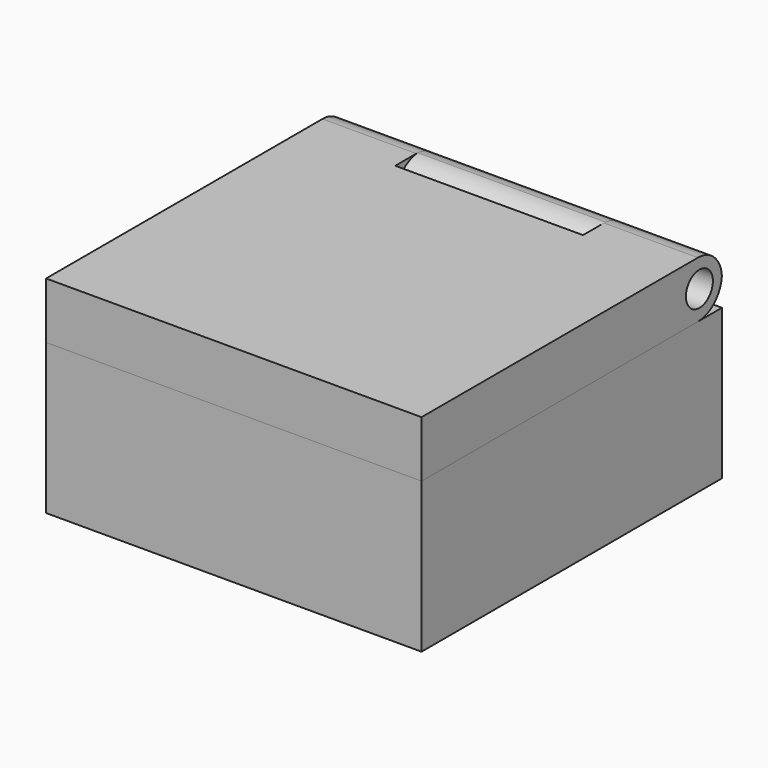
from build123d import *

# Parameters (mm, degrees)
F0_W        = 25.4
F0_H        = 25.4
F1_DEPTH    = 10.16
F2_W        = 17.78
F2_H        = 17.78
F3_DEPTH    = 5.08
F4_W        = 6.35
F4_H        = 3.81
F5_DEPTH    = 3.81
F7_DEPTH    = 3.81
F8_T1_DEPTH = 16.51
F8_T3_DEPTH = 16.51
F9_T1_DEPTH = 22.86
F10_R       = 1.1410136833
F11_DEPTH   = 25.4


# Not quite as in the source:
# - a fillet or chamfer that OpenCascade refuses, or shapes differently, is made with other operations: its cross-section is extruded or revolved along the edge and cut away or added


with BuildPart() as f1:
    # F0 (on Top) → F1 (new body)
    with BuildSketch(Plane.XY):
        with Locations((12.7, 12.7)):
            Rectangle(F0_W, F0_H)
    extrude(amount=F1_DEPTH)

    # F2 (on face) → F3 (cut)
    with BuildSketch(Plane.XY.offset(10.16)):
        with Locations((12.7, 12.7)):
            Rectangle(F2_W, F2_H)
    extrude(amount=-F3_DEPTH, mode=Mode.SUBTRACT)

    # F4 (on face) → F5 (join)
    with BuildSketch(Plane.XY.offset(10.16)):
        with Locations((9.525, 23.495)):
            Rectangle(F4_W, F4_H)
        with Locations((15.875, 23.495)):
            Rectangle(F4_W, F4_H)
    extrude(amount=F5_DEPTH)

    # F9: fillet of radius 2.032 on 2 edges, made by hand

    # F9_s2 → F9_t1 (cut)
    with BuildSketch(Plane.YZ.offset(1.27)):
        with BuildLine():
            ThreePointArc((21.59, 11.938), (22.1851590206, 13.3748409794), (23.622, 13.97))
            Line((23.622, 13.97), (21.59, 13.97))
            Line((21.59, 13.97), (21.59, 11.938))
        make_face()
        with BuildLine():
            ThreePointArc((25.4, 11.938), (24.8048409794, 13.3748409794), (23.368, 13.97))
            Line((23.368, 13.97), (25.4, 13.97))
            Line((25.4, 13.97), (25.4, 11.938))
        make_face()
    extrude(amount=F9_T1_DEPTH, mode=Mode.SUBTRACT)


with BuildPart() as f7:
    # F6 (on face) → F7 (new body)
    with BuildSketch(Plane.XY.offset(10.16)):
        Polygon((3.81, 21.59), (0, 21.59), (0, 0), (25.4, 0), (25.4, 21.59), (21.59, 21.59), (21.59, 3.81), (3.81, 3.81), align=None)
        Polygon((6.35, 21.59), (3.81, 21.59), (3.81, 3.81), (21.59, 3.81), (21.59, 21.59), (19.05, 21.59), align=None)
        Polygon((19.05, 25.4), (19.05, 21.59), (21.59, 21.59), (25.4, 21.59), (25.4, 25.4), align=None)
        Polygon((0, 25.4), (0, 21.59), (3.81, 21.59), (6.35, 21.59), (6.35, 25.4), align=None)
    extrude(amount=F7_DEPTH)

    # F8: fillet of radius 2.032 on 4 edges, made by hand

    # F8_s2 → F8_t1 (cut)
    with BuildSketch(Plane.YZ.offset(-5.08)):
        with BuildLine():
            ThreePointArc((25.4, 12.192), (24.8048409794, 10.7551590206), (23.368, 10.16))
            Line((23.368, 10.16), (25.4, 10.16))
            Line((25.4, 10.16), (25.4, 12.192))
        make_face()
        with BuildLine():
            ThreePointArc((25.4, 11.938), (24.8048409794, 13.3748409794), (23.368, 13.97))
            Line((23.368, 13.97), (25.4, 13.97))
            Line((25.4, 13.97), (25.4, 11.938))
        make_face()
    extrude(amount=F8_T1_DEPTH, mode=Mode.SUBTRACT)

    # F8_s4 → F8_t3 (cut)
    with BuildSketch(Plane.YZ.offset(13.97)):
        with BuildLine():
            ThreePointArc((25.4, 11.938), (24.8048409794, 13.3748409794), (23.368, 13.97))
            Line((23.368, 13.97), (25.4, 13.97))
            Line((25.4, 13.97), (25.4, 11.938))
        make_face()
        with BuildLine():
            ThreePointArc((25.4, 12.192), (24.8048409794, 10.7551590206), (23.368, 10.16))
            Line((23.368, 10.16), (25.4, 10.16))
            Line((25.4, 10.16), (25.4, 12.192))
        make_face()
    extrude(amount=F8_T3_DEPTH, mode=Mode.SUBTRACT)


with BuildPart() as f11_tool:
    # F10 (on face) → F11 (new body)
    with BuildSketch(Plane.YZ.offset(25.4)):
        with Locations((23.495, 12.0630136833)):
            Circle(F10_R)
    extrude(amount=-F11_DEPTH)


with BuildPart() as f1_1:
    add(f1.part)

    # F11: cut by f11_tool
    add(f11_tool.part, mode=Mode.SUBTRACT)


with BuildPart() as f7_1:
    add(f7.part)

    # F11: cut by f11_tool
    add(f11_tool.part, mode=Mode.SUBTRACT)


solid = Compound([f1_1.part, f7_1.part])
